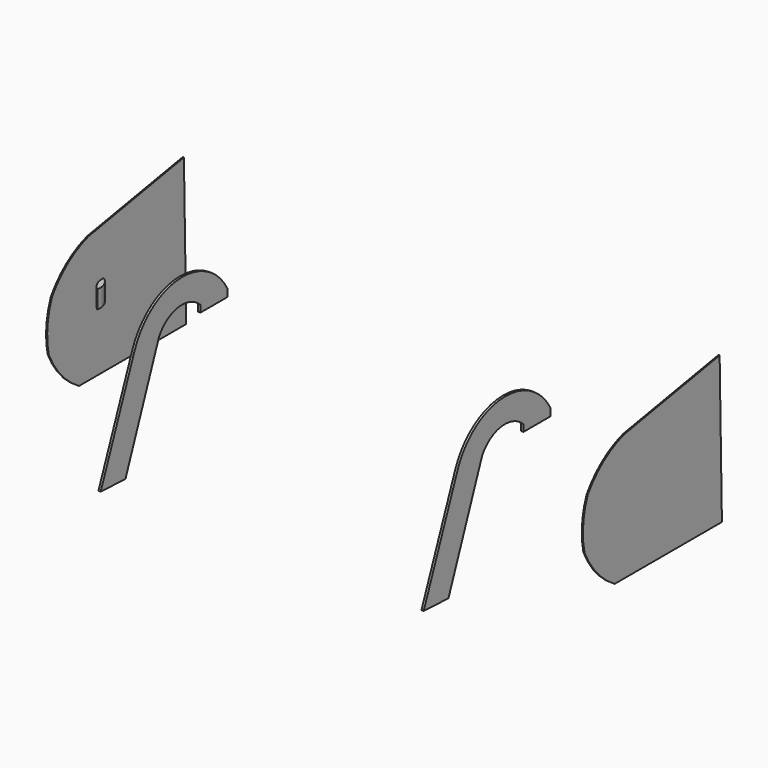
from build123d import *

# Parameters (mm, degrees)
F3_DEPTH  = 12.7
F8_DEPTH  = 0.79375
F12_DEPTH = 1.5875


# Not quite as in the source:
# - a feature names something its author has since deleted; it is built from what else it names
# - the program builds the solid bodies; features that only make, move or delete a surface that nothing else refers to are left out


with BuildPart() as f3:
    # F2 (on Top) → F3 (new body)
    with BuildSketch(Plane.XY):
        with BuildLine():
            ThreePointArc((10.8289094642, -43.4034839272), (9.8562802874, -36.1129352639), (5.002938211, -30.5863469839))
            ThreePointArc((5.002938211, -30.5863469839), (6.2969861268, -37.7307962225), (10.8289094642, -43.4034839272))
        make_face()
    extrude(amount=F3_DEPTH)


with BuildPart() as f3_1:
    # F4: moved
    add(f3.part.moved(Location((0, 0, -15.24))))


with BuildPart() as f3_2:
    # F5: moved
    add(f3_1.part.moved(Location((-190.5, 0, 0))))


with BuildPart() as f6_1:
    # F6: instance of F3
    add(f3_2.part.mirror(Plane.YZ))


with BuildPart() as f8:
    # F7 (on Right) → F8 (new body)
    with BuildSketch(Plane.YZ):
        with BuildLine():
            Line((49.2759980261, -65.5319988728), (47.2440011799, 39.8779995739))
            Line((47.2440011799, 39.8779995739), (-37.8459990025, 24.8920004815))
            ThreePointArc((-37.8459990025, 24.8920004815), (-56.3244526147, 15.3487957848), (-70.3580006957, 0))
            ThreePointArc((-70.3580006957, 0), (-74.3783630308, -17.3168922416), (-73.1519982219, -35.0520014763))
            ThreePointArc((-73.1519982219, -35.0520014763), (-62.0472133534, -52.3742066317), (-46.2279990315, -65.5319988728))
            Line((-46.2279990315, -65.5319988728), (49.2759980261, -65.5319988728))
        make_face()
    extrude(amount=F8_DEPTH)


with BuildPart() as f8_1:
    # F9: moved
    add(f8.part.moved(Location((190.5, 0, 0))))


with BuildPart() as f10_1:
    # F10: instance of F8
    add(f8_1.part.mirror(Plane.YZ))


with BuildPart() as f12:
    # F11 (on Right) → F12 (new body)
    with BuildSketch(Plane.YZ):
        with BuildLine():
            Line((-33.2739986479, 4.8797923156), (-33.2739986479, 0))
            Line((-33.2739986479, 0), (-9.1439997777, 0))
            Line((-9.1439997777, 0), (-9.1439997777, 5.2811519084))
            ThreePointArc((-9.1439997777, 5.2811519084), (-52.2189865365, 28.8715738057), (-91.9480025768, 0))
            Line((-91.9480025768, 0), (-122.1739947796, -76.2000009418))
            Line((-122.1739947796, -76.2000009418), (-100.0759974122, -77.2159993649))
            Line((-100.0759974122, -77.2159993649), (-70.1040029526, 0))
            ThreePointArc((-70.1040029526, 0), (-52.8795005415, 11.4251372829), (-33.2739986479, 4.8797923156))
        make_face()
    extrude(amount=F12_DEPTH)


with BuildPart() as f12_1:
    # F13: moved
    add(f12.part.moved(Location((114.3, 0, 0))))


with BuildPart() as f14_1:
    # F14: instance of F12
    add(f12_1.part.mirror(Plane.YZ))


solid = Compound([f3_2.part, f6_1.part, f8_1.part, f10_1.part, f12_1.part, f14_1.part])
